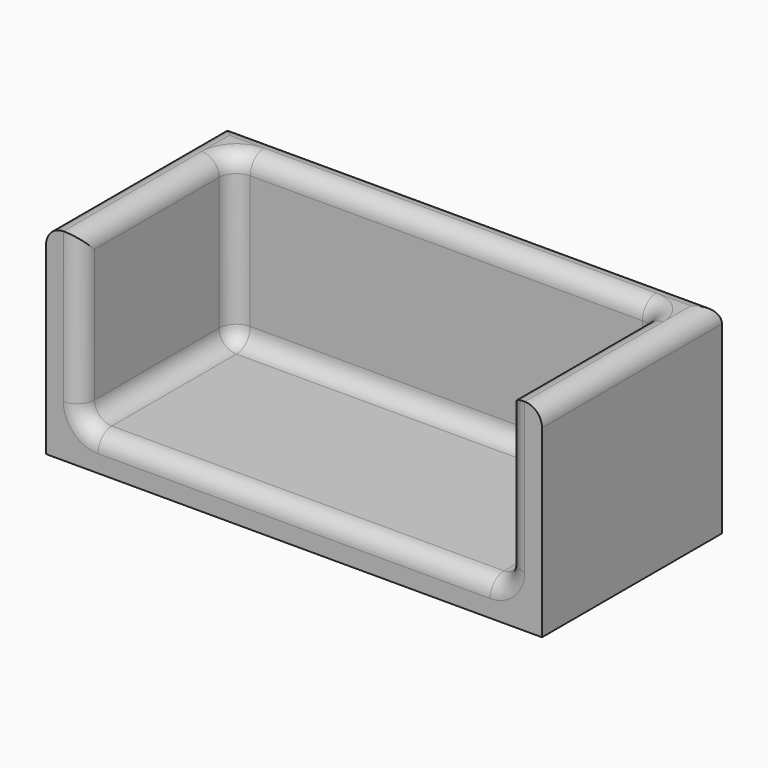
from build123d import *

# Parameters (mm, degrees)
F0_W     = 2184.4
F0_H     = 990.6
F1_DEPTH = 889
F2_T     = -152.4
F3_R     = 76.2
F4_R     = 76.19999


# Not quite as in the source:
# - a fillet or chamfer is up to 0.001 mm smaller than in the source, because OpenCascade refuses the exact size


with BuildPart() as f1:
    # F0 (on Top) → F1 (new body)
    with BuildSketch(Plane.XY):
        with Locations((2.5491379201, 53.3265618357)):
            Rectangle(F0_W, F0_H)
    extrude(amount=F1_DEPTH)

    # F2
    f2_openings = [f1.faces().sort_by_distance(p)[0] for p in [
        (2.549138, 53.326562, 889),
        (2.549138, -441.973438, 444.5),
    ]]
    offset(amount=F2_T, openings=f2_openings)

    # F3
    f3_edges = [f1.edges().sort_by_distance(p)[0] for p in [
        (2.549138, 396.226562, 889),
        (-937.250862, 396.226562, 520.7),
        (2.549138, 396.226562, 152.4),
        (942.349138, 396.226562, 520.7),
        (2.549138, -441.973438, 152.4),
        (942.349138, -22.873438, 152.4),
        (-937.250862, -22.873438, 152.4),
        (-937.250862, -441.973438, 520.7),
        (-937.250862, -22.873438, 889),
        (942.349138, -441.973438, 520.7),
        (942.349138, -22.873438, 889),
    ]]
    fillet(f3_edges, radius=F3_R)

    # F4 (radius 76.2 in the source; OpenCascade refuses exactly that, so slightly less here)
    f4_edges = [f1.edges().sort_by_distance(p)[0] for p in [
        (1094.749138, 53.326562, 889),
        (2.549138, 548.626562, 889),
        (-1089.650862, 53.326562, 889),
    ]]
    fillet(f4_edges, radius=F4_R)


solid = f1.part
